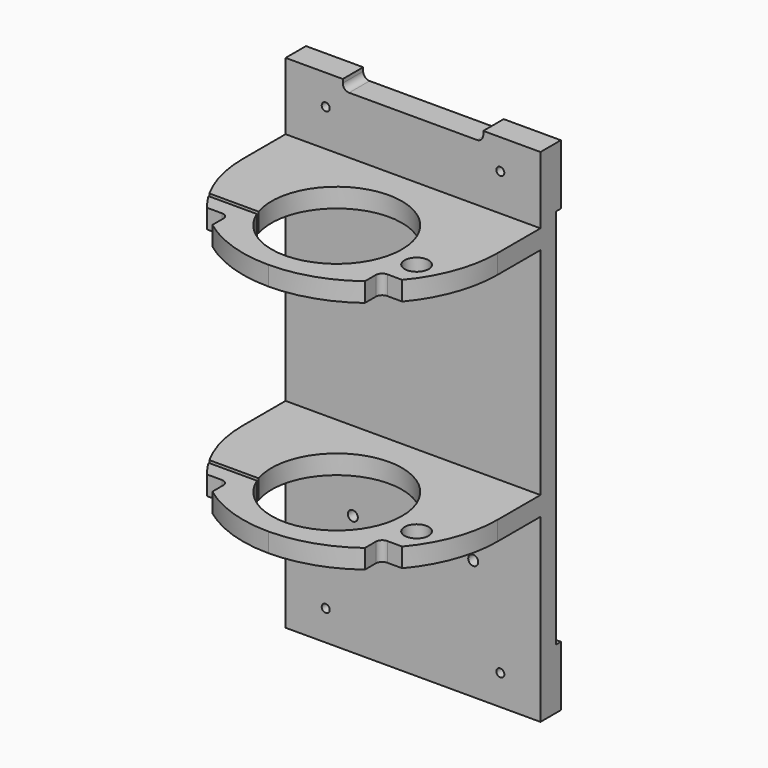
from build123d import *

# Parameters (mm, degrees)
F0_W     = 127
F0_H     = 30
F0_H_2   = 190
F1_DEPTH = 9.53
F2_DEPTH = 3.18
F4_D     = 4
F5_D     = 5
F3_W     = 127
F3_H     = 9.53
F6_DEPTH = 90.12
F8_DEPTH = 216.521
F9_D     = 12
F10_R    = 3.175


with BuildPart() as f1:
    # F0 (on Front) → F1 (new body)
    with BuildSketch(Plane.XZ):
        with Locations((0, -110)):
            Rectangle(F0_W, F0_H)
        Rectangle(F0_W, F0_H_2)
        Polygon((-63.5, 95), (63.5, 95), (63.5, 125), (35, 125), (35, 120), (-35, 120), (-35, 125), (-63.5, 125), align=None)
    extrude(amount=F1_DEPTH)

    # F0 (on Front) → F2 (join)
    with BuildSketch(Plane.XZ):
        Polygon((-63.5, 95), (63.5, 95), (63.5, 125), (35, 125), (35, 120), (-35, 120), (-35, 125), (-63.5, 125), align=None)
        with Locations((0, -110)):
            Rectangle(F0_W, F0_H)
    extrude(amount=-F2_DEPTH)

    # F4 (through all)
    with Locations(Plane.XZ.offset(9.53)):
        with Locations((-43.5, 110), (43.5, 110), (-43.5, -110), (43.5, -110)):
            Hole(F4_D / 2)

    # F5 (through all)
    with Locations(Plane(origin=(0, 0, 0), x_dir=(1, 0, 0), z_dir=(0, 1, 0))):
        with Locations((-30, 65), (30, 65)):
            Hole(F5_D / 2)

    # F3 (on face) → F6 (join)
    with BuildSketch(Plane.XZ.offset(9.53)):
        with Locations((0, 86.755)):
            Rectangle(F3_W, F3_H)
        with Locations((0, -30.235)):
            Rectangle(F3_W, F3_H)
    extrude(amount=F6_DEPTH)

    # F7 (on face) → F8 (cut, through all)
    with BuildSketch(Plane.XY.offset(91.52)):
        with BuildLine():
            Line((-30.2034766211, -69.03), (-30.9232921921, -67.03))
            ThreePointArc((-30.9232921921, -67.03), (-30.5797394754, -68.0358863166), (-30.2034766211, -69.03))
        make_face()
        with BuildLine():
            ThreePointArc((-30.2034766211, -69.03), (6.1088873707, -88.9507063689), (32.5, -57.03))
            ThreePointArc((32.5, -57.03), (-5.0617686512, -24.9265967829), (-30.9232921921, -67.03))
            Line((-30.9232921921, -67.03), (-30.2034766211, -69.03))
        make_face()
        with BuildLine():
            ThreePointArc((-54.3245395747, -69.03), (-54.9142828433, -68.0352871997), (-55.4858144033, -67.03))
            ThreePointArc((-55.4858144033, -67.03), (-61.4638072959, -52.1015012677), (-63.5, -36.15))
            Line((-63.5, -36.15), (-63.5, -99.65))
            Line((-63.5, -99.65), (2.176e-07, -99.65))
            ThreePointArc((2.176e-07, -99.65), (-20.0212042966, -96.4111100007), (-38, -87.0248464371))
            ThreePointArc((-38, -87.0248464371), (-43.5829123177, -82.3320284732), (-48.5909003827, -77.03))
            ThreePointArc((-48.5909003827, -77.03), (-51.6129532715, -73.1412564614), (-54.3245395747, -69.03))
        make_face()
        with BuildLine():
            ThreePointArc((38, -87.0248464371), (20.0212045031, -96.4111099321), (2.176e-07, -99.65))
            Line((2.176e-07, -99.65), (63.5, -99.65))
            Line((63.5, -99.65), (63.5, -36.15))
            ThreePointArc((63.5, -36.15), (59.6564002195, -57.9069279277), (48.5909003827, -77.03))
            ThreePointArc((48.5909003827, -77.03), (43.5829123177, -82.3320284732), (38, -87.0248464371))
        make_face()
        with BuildLine():
            Line((-38, -77.03), (-48.5909003827, -77.03))
            ThreePointArc((-48.5909003827, -77.03), (-43.5829123177, -82.3320284732), (-38, -87.0248464371))
            Line((-38, -87.0248464371), (-38, -77.03))
        make_face()
        with BuildLine():
            Line((38, -77.03), (38, -87.0248464371))
            ThreePointArc((38, -87.0248464371), (43.5829123177, -82.3320284732), (48.5909003827, -77.03))
            Line((48.5909003827, -77.03), (38, -77.03))
        make_face()
        with BuildLine():
            ThreePointArc((-30.2034766211, -69.03), (-30.5797394754, -68.0358863166), (-30.9232921921, -67.03))
            Line((-30.9232921921, -67.03), (-55.4858144033, -67.03))
            ThreePointArc((-55.4858144033, -67.03), (-54.9142828433, -68.0352871997), (-54.3245395747, -69.03))
            Line((-54.3245395747, -69.03), (-30.2034766211, -69.03))
        make_face()
    extrude(amount=-F8_DEPTH, mode=Mode.SUBTRACT)

    # F9 (through all)
    with Locations(Plane.XY.offset(91.52)):
        with Locations((45, -63.53)):
            Hole(F9_D / 2)

    # F10
    f10_edges = [f1.edges().sort_by_distance(p)[0] for p in [
        (-38, -77.03, 86.755),
        (-38, -77.03, -30.235),
        (38, -77.03, -30.235),
        (38, -77.03, 86.755),
        (-35, -3.175, 120),
        (35, -3.175, 120),
    ]]
    fillet(f10_edges, radius=F10_R)


solid = f1.part
